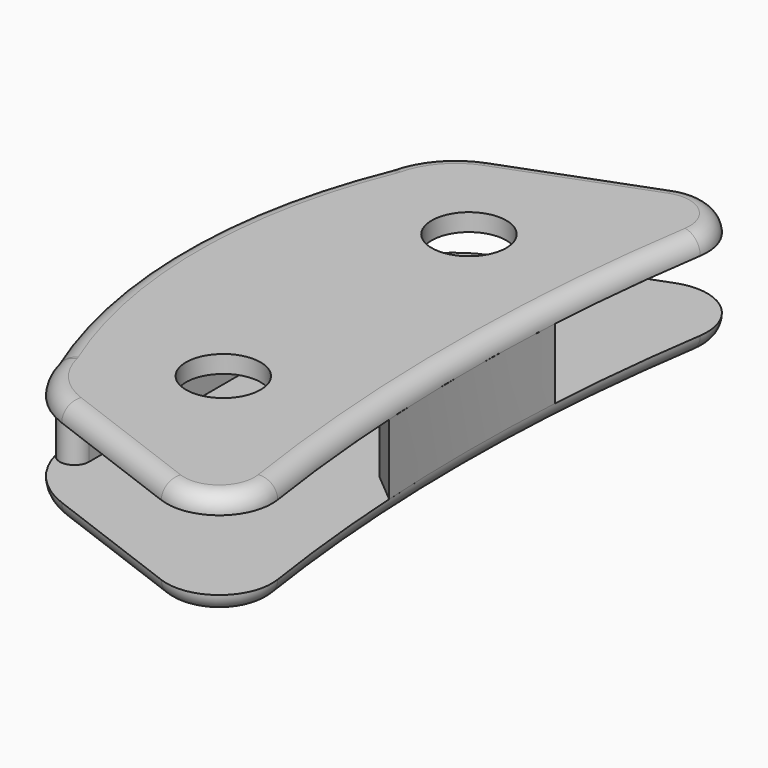
from build123d import *

# Parameters (mm, degrees)
F1_DEPTH  = 2
F2_R      = 5.6
F3_DEPTH  = 1.5
F5_DEPTH  = 10
F7_DEPTH  = 2
F8_R      = 1.99999
F9_R      = 4.25
F10_DEPTH = 2


# Not quite as in the source:
# - a fillet or chamfer is up to 0.001 mm smaller than in the source, because OpenCascade refuses the exact size


with BuildPart() as f1:
    # F0 (on Top) → F1 (new body)
    with BuildSketch(Plane.XY):
        with BuildLine():
            Line((8.2361189543, 36.6168409437), (-7.9935965644, 30.5207371811))
            ThreePointArc((-7.9935965644, 30.5207371811), (-11.9662543406, 27.7862465208), (-14.1970285873, 23.510372898))
            ThreePointArc((-14.1970285873, 23.510372898), (-17, 0), (-14.1970285873, -23.510372898))
            ThreePointArc((-14.1970285873, -23.510372898), (-11.9662543406, -27.7862465208), (-7.9935965644, -30.5207371811))
            Line((-7.9935965644, -30.5207371811), (8.2361189543, -36.6168409437))
            ThreePointArc((8.2361189543, -36.6168409437), (14.1245779615, -35.6606279318), (16.2775548115, -30.0970873786))
            ThreePointArc((16.2775548115, -30.0970873786), (14, 0), (16.2775548115, 30.0970873786))
            ThreePointArc((16.2775548115, 30.0970873786), (14.1245779615, 35.6606279318), (8.2361189543, 36.6168409437))
        make_face()
    extrude(amount=F1_DEPTH)

    # F2 (on face) → F3 (cut)
    with BuildSketch(Plane.XY.offset(2)):
        with Locations((0, 17.5)):
            Circle(F2_R)
        with Locations((0, -17.5)):
            Circle(F2_R)
    extrude(amount=-F3_DEPTH, mode=Mode.SUBTRACT)

    # F4 (on Top) → F5 (join)
    with BuildSketch(Plane.XY):
        with BuildLine():
            Line((-11, -22.8789469535), (-11, 22.8789469535))
            ThreePointArc((-11, 22.8789469535), (-12.3390571638, 24.5083402847), (-14.1970285873, 23.510372898))
            ThreePointArc((-14.1970285873, 23.510372898), (-18.8404213522, 0), (-14.1970285873, -23.510372898))
            ThreePointArc((-14.1970285873, -23.510372898), (-12.3390571638, -24.5083402847), (-11, -22.8789469535))
        make_face()
        with BuildLine():
            Line((14.3490034732, 11.8101475791), (11, 9))
            Line((11, 9), (11, -9))
            Line((11, -9), (14.3490034732, -11.8101475791))
            ThreePointArc((14.3490034732, -11.8101475791), (14, 0), (14.3490034732, 11.8101475791))
        make_face()
    extrude(amount=F5_DEPTH)

    # F6 (on face) → F7 (join)
    with BuildSketch(Plane.XY.offset(10)):
        with BuildLine():
            Line((8.2361189543, 36.6168409437), (-7.9935965644, 30.5207371811))
            ThreePointArc((-7.9935965644, 30.5207371811), (-11.9662543406, 27.7862465208), (-14.1970285873, 23.510372898))
            ThreePointArc((-14.1970285873, 23.510372898), (-12.3390571638, 24.5083402847), (-11, 22.8789469535))
            Line((-11, 22.8789469535), (-11, -22.8789469535))
            ThreePointArc((-11, -22.8789469535), (-12.3390571638, -24.5083402847), (-14.1970285873, -23.510372898))
            ThreePointArc((-14.1970285873, -23.510372898), (-11.9662543406, -27.7862465208), (-7.9935965644, -30.5207371811))
            Line((-7.9935965644, -30.5207371811), (8.2361189543, -36.6168409437))
            ThreePointArc((8.2361189543, -36.6168409437), (14.1245779615, -35.6606279318), (16.2775548115, -30.0970873786))
            ThreePointArc((16.2775548115, -30.0970873786), (14, 0), (16.2775548115, 30.0970873786))
            ThreePointArc((16.2775548115, 30.0970873786), (14.1245779615, 35.6606279318), (8.2361189543, 36.6168409437))
        make_face()
        with BuildLine():
            ThreePointArc((-11, 22.8789469535), (-12.3390571638, 24.5083402847), (-14.1970285873, 23.510372898))
            ThreePointArc((-14.1970285873, 23.510372898), (-18.8404213522, 0), (-14.1970285873, -23.510372898))
            ThreePointArc((-14.1970285873, -23.510372898), (-12.3390571638, -24.5083402847), (-11, -22.8789469535))
            Line((-11, -22.8789469535), (-11, 22.8789469535))
        make_face()
    extrude(amount=F7_DEPTH)

    # F8 (radius 2 in the source; OpenCascade refuses exactly that, so slightly less here)
    f8_edges = [f1.edges().sort_by_distance(p)[0] for p in [
        (14.124578, 35.660628, 12),
        (0.121261, 33.568789, 12),
        (-11.966254, 27.786247, 12),
        (-18.840421, 0, 12),
        (-11.966254, -27.786247, 12),
        (0.121261, -33.568789, 12),
        (14.124578, -35.660628, 12),
        (14, 0, 12),
        (-18.840421, 0, 0),
        (14, 0, 0),
    ]]
    fillet(f8_edges, radius=F8_R)

    # F9 (on face) → F10 (cut)
    with BuildSketch(Plane(origin=(0, 0, 10), x_dir=(1, 0, 0), z_dir=(0, 0, -1))):
        with Locations((0, 17.5)):
            Circle(F9_R)
        with Locations((0, -17.5)):
            Circle(F9_R)
    extrude(amount=-F10_DEPTH, mode=Mode.SUBTRACT)


solid = f1.part
